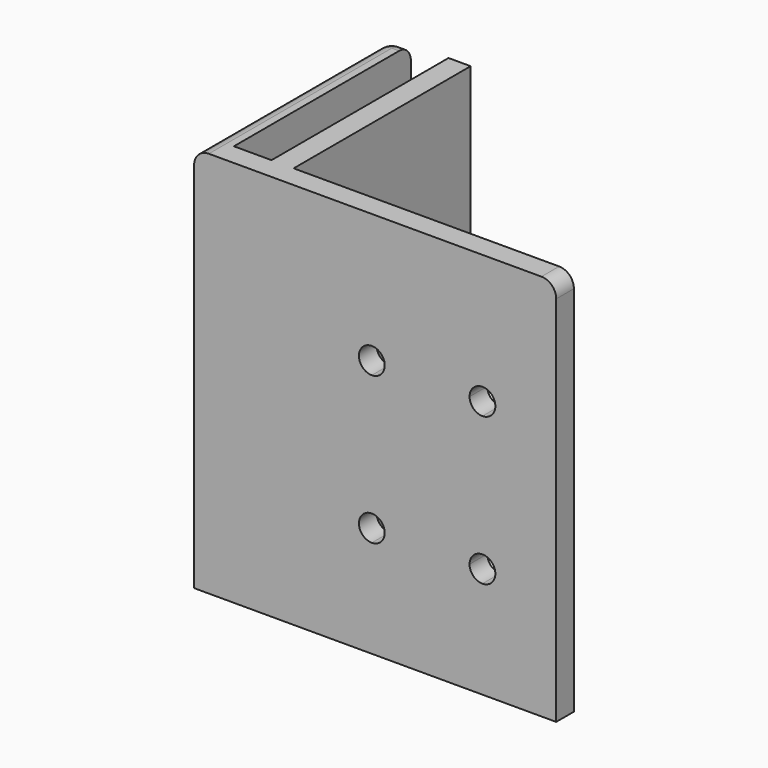
from build123d import *

# Parameters (mm, degrees)
F0_W     = 3
F0_H     = 30
F1_DEPTH = 52.5
F3_DEPTH = 25
F4_R     = 2
F6_DEPTH = 25


# Not quite as in the source:
# - a feature names something its author has since deleted; it is built from what else it names


with BuildPart() as f1:
    # F0 (on Top) → F1 (new body)
    with BuildSketch(Plane.XY):
        Polygon((2, 0), (-1, 0), (-6.1, 0), (-6.1, 30), (-9.1, 30), (-9.1, -2.9952730983), (40, -3), (40, 0), align=None)
        with Locations((0.5, 15)):
            Rectangle(F0_W, F0_H)
    extrude(amount=F1_DEPTH)

    # F2 (on face) → F3 (cut)
    with BuildSketch(Plane(origin=(-9.1, 0, 0), x_dir=(0, -1, 0), z_dir=(-1, 0, 0))):
        with BuildLine():
            Line((-13.5023634508, 37.5), (-13.5023634508, 39.25))
            ThreePointArc((-13.5023634508, 39.25), (-15.2523634508, 37.5), (-13.5023634508, 35.75))
            Line((-13.5023634508, 35.75), (-13.5023634508, 37.5))
        make_face()
        with BuildLine():
            ThreePointArc((-11.7523634508, 37.5), (-12.2649265837, 38.7374368671), (-13.5023634508, 39.25))
            Line((-13.5023634508, 39.25), (-13.5023634508, 37.5))
            Line((-13.5023634508, 37.5), (-13.5023634508, 35.75))
            ThreePointArc((-13.5023634508, 35.75), (-12.2649265837, 36.2625631329), (-11.7523634508, 37.5))
        make_face()
        with BuildLine():
            Line((-13.5023634508, 15), (-13.5023634508, 13.25))
            ThreePointArc((-13.5023634508, 13.25), (-12.2649265837, 13.7625631329), (-11.7523634508, 15))
            ThreePointArc((-11.7523634508, 15), (-12.2649265837, 16.2374368671), (-13.5023634508, 16.75))
            Line((-13.5023634508, 16.75), (-13.5023634508, 15))
        make_face()
        with BuildLine():
            ThreePointArc((-13.5023634508, 16.75), (-15.2523634508, 15), (-13.5023634508, 13.25))
            Line((-13.5023634508, 13.25), (-13.5023634508, 15))
            Line((-13.5023634508, 15), (-13.5023634508, 16.75))
        make_face()
    extrude(amount=-F3_DEPTH, mode=Mode.SUBTRACT)

    # F4
    f4_edges = [f1.edges().sort_by_distance(p)[0] for p in [
        (40, -1.5, 52.5),
        (-9.1, 30, 26.25),
        (-9.1, 13.502363, 52.5),
        (-7.6, 30, 52.5),
    ]]
    fillet(f4_edges, radius=F4_R)

    # F5 (on face) → F6 (cut)
    with BuildSketch(Plane(origin=(-0.000288442, -2.9961491359, 0), x_dir=(0.9999999954, -9.62709e-05, 0), z_dir=(-9.62709e-05, -0.9999999954, 0))):
        with BuildLine():
            Line((15.0002886274, 35), (15.0002886274, 33.25))
            ThreePointArc((15.0002886274, 33.25), (16.2377254944, 33.7625631329), (16.7502886274, 35))
            Line((16.7502886274, 35), (15.0002886274, 35))
        make_face()
        with BuildLine():
            ThreePointArc((15.0002886274, 36.75), (13.2502886274, 35), (15.0002886274, 33.25))
            Line((15.0002886274, 33.25), (15.0002886274, 35))
            Line((15.0002886274, 35), (15.0002886274, 36.75))
        make_face()
        with BuildLine():
            Line((15.0002886274, 36.75), (15.0002886274, 35))
            Line((15.0002886274, 35), (16.7502886274, 35))
            ThreePointArc((16.7502886274, 35), (16.2377254944, 36.2374368671), (15.0002886274, 36.75))
        make_face()
        with BuildLine():
            Line((30.0002886274, 35), (31.7502886274, 35))
            ThreePointArc((31.7502886274, 35), (31.2377254944, 36.2374368671), (30.0002886274, 36.75))
            Line((30.0002886274, 36.75), (30.0002886274, 35))
        make_face()
        with BuildLine():
            Line((28.2502886274, 35), (30.0002886274, 35))
            Line((30.0002886274, 35), (30.0002886274, 36.75))
            ThreePointArc((30.0002886274, 36.75), (28.7628517603, 36.2374368671), (28.2502886274, 35))
        make_face()
        with BuildLine():
            Line((30.0002886274, 33.25), (30.0002886274, 35))
            Line((30.0002886274, 35), (28.2502886274, 35))
            ThreePointArc((28.2502886274, 35), (28.7628517603, 33.7625631329), (30.0002886274, 33.25))
        make_face()
        with BuildLine():
            ThreePointArc((30.0002886274, 33.25), (31.2377254944, 33.7625631329), (31.7502886274, 35))
            Line((31.7502886274, 35), (30.0002886274, 35))
            Line((30.0002886274, 35), (30.0002886274, 33.25))
        make_face()
        with BuildLine():
            Line((30.0002886274, 15), (31.7502886274, 15))
            ThreePointArc((31.7502886274, 15), (31.2377254944, 16.2374368671), (30.0002886274, 16.75))
            Line((30.0002886274, 16.75), (30.0002886274, 15))
        make_face()
        with BuildLine():
            Line((28.2502886274, 15), (30.0002886274, 15))
            Line((30.0002886274, 15), (30.0002886274, 16.75))
            ThreePointArc((30.0002886274, 16.75), (28.7628517603, 16.2374368671), (28.2502886274, 15))
        make_face()
        with BuildLine():
            ThreePointArc((28.2502886274, 15), (28.7628517603, 13.7625631329), (30.0002886274, 13.25))
            Line((30.0002886274, 13.25), (30.0002886274, 15))
            Line((30.0002886274, 15), (28.2502886274, 15))
        make_face()
        with BuildLine():
            Line((30.0002886274, 15), (30.0002886274, 13.25))
            ThreePointArc((30.0002886274, 13.25), (31.2377254944, 13.7625631329), (31.7502886274, 15))
            Line((31.7502886274, 15), (30.0002886274, 15))
        make_face()
        with BuildLine():
            Line((15.0002886274, 15), (15.0002886274, 13.25))
            ThreePointArc((15.0002886274, 13.25), (16.2377254944, 13.7625631329), (16.7502886274, 15))
            Line((16.7502886274, 15), (15.0002886274, 15))
        make_face()
        with BuildLine():
            Line((15.0002886274, 16.75), (15.0002886274, 15))
            Line((15.0002886274, 15), (16.7502886274, 15))
            ThreePointArc((16.7502886274, 15), (16.2377254944, 16.2374368671), (15.0002886274, 16.75))
        make_face()
        with BuildLine():
            ThreePointArc((15.0002886274, 16.75), (13.2502886274, 15), (15.0002886274, 13.25))
            Line((15.0002886274, 13.25), (15.0002886274, 15))
            Line((15.0002886274, 15), (15.0002886274, 16.75))
        make_face()
    extrude(amount=-F6_DEPTH, mode=Mode.SUBTRACT)


solid = f1.part
